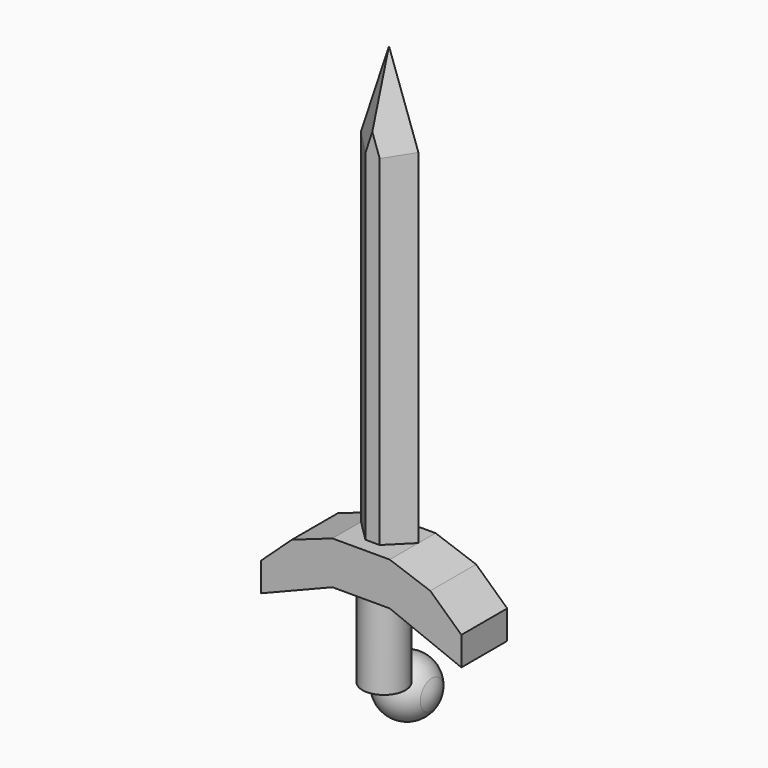
from build123d import *

# Parameters (mm, degrees)
F1_DEPTH = 20
F0_W     = 20
F0_H     = 120
F2_DEPTH = 15
F3_SIZE  = 7.49999
F5_R     = 7.5
F6_DEPTH = 30


# Not quite as in the source:
# - a fillet or chamfer is up to 0.001 mm smaller than in the source, because OpenCascade refuses the exact size


with BuildPart() as f1:
    # F0 (on Front) → F1 (new body)
    with BuildSketch(Plane.XZ):
        Polygon((-23.8778254464, 10.0028783713), (-34.7346724942, 0), (-9.7346724942, 0), (10.2653275058, 0), (35.2653275058, 0), (24.4084804579, 10.0028783713), (10.2653275058, 15), (-9.7346724942, 15), align=None)
        Polygon((-9.7346724942, 0), (-34.7346724942, 0), (-34.7346724942, -10), align=None)
        Polygon((35.2653275058, 0), (10.2653275058, 0), (35.2653275058, -10), align=None)
    extrude(amount=F1_DEPTH)

    # F5 (on face) → F6 (join)
    with BuildSketch(Plane(origin=(0, 0, 0), x_dir=(1, 0, 0), z_dir=(0, 0, -1))):
        with Locations((0.2653275058, 10)):
            Circle(F5_R)
    extrude(amount=F6_DEPTH)


with BuildPart() as f2:
    # F0 (on Front) → F2 (new body)
    with BuildSketch(Plane.XZ):
        with Locations((0.2653275058, 75)):
            Rectangle(F0_W, F0_H)
        Polygon((0, 164.3196642399), (-9.7346724942, 135), (10.2653275058, 135), align=None)
    extrude(amount=F2_DEPTH)

    # F3 (size 7.5 in the source; OpenCascade refuses exactly that, so slightly less here)
    f3_edges = [f2.edges().sort_by_distance(p)[0] for p in [
        (-9.734672, -15, 75),
        (-9.734672, 0, 75),
        (10.265328, 0, 75),
        (10.265328, -15, 75),
        (5.132664, 0, 149.659832),
        (5.132664, -15, 149.659832),
        (-4.867336, -15, 149.659832),
        (-4.867336, 0, 149.659832),
    ]]
    chamfer(f3_edges, length=F3_SIZE)


with BuildPart() as f4:
    # F0 (on Front) → F4 (revolve)
    with BuildSketch(Plane.XZ):
        with BuildLine():
            Line((8.9255815436, -30), (-8.3949265321, -30))
            ThreePointArc((-8.3949265321, -30), (-9.3939307571, -32.411809549), (-9.7346724942, -35))
            Line((-9.7346724942, -35), (10.2653275058, -35))
            ThreePointArc((10.2653275058, -35), (9.9245857687, -32.411809549), (8.9255815436, -30))
        make_face()
        with BuildLine():
            ThreePointArc((8.9255815436, -30), (0.2653275058, -25), (-8.3949265321, -30))
            Line((-8.3949265321, -30), (8.9255815436, -30))
        make_face()
    revolve(axis=Axis((0.2653275058, 0, -35), (1, 0, 0)))


solid = Compound([f1.part, f2.part, f4.part])
